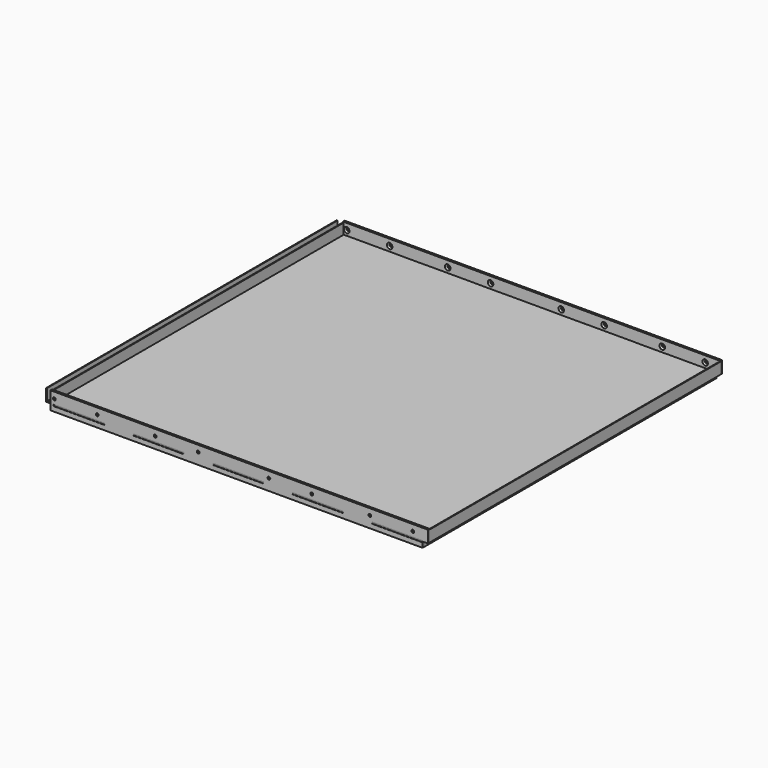
from build123d import *

# Parameters (mm, degrees)
F1_DEPTH        = 1440
F2_DEPTH        = 1440
F3_W            = 200
F3_H            = 7
F4_DEPTH        = 3
F5_W            = 200
F5_H            = 7
F6_DEPTH        = 3
F7_W            = 200.5
F7_H            = 6.5
F8_DEPTH        = 8
F11_D           = 11
F11_CSINK_D     = 22
F11_CSINK_ANGLE = 90


with BuildPart() as f1:
    # F0 (on Front) → F1 (new body)
    with BuildSketch(Plane.XZ):
        Polygon((-1400.4856245518, 88.2625505924), (-1403.4856245518, 88.2625505924), (-1403.4856245518, 40.2625505924), (91.5143754482, 40.2625505924), (91.5143754482, 21.2625505924), (94.5143754482, 21.2625505924), (94.5143754482, 43.2625505924), (-1379.4856245518, 43.2625505924), (-1400.4856245518, 43.2625505924), align=None)
    extrude(amount=-F1_DEPTH)

    # F3 (on face) → F4 (join)
    with BuildSketch(Plane.XY.offset(43.2625505924)):
        with Locations((-1266.4856245518, -3.5)):
            Rectangle(F3_W, F3_H)
        with Locations((-951.4856245518, -3.5)):
            Rectangle(F3_W, F3_H)
        with Locations((-636.4856245518, -3.5)):
            Rectangle(F3_W, F3_H)
        with Locations((-321.4856245518, -3.5)):
            Rectangle(F3_W, F3_H)
        with Locations((-6.4856245518, -3.5)):
            Rectangle(F3_W, F3_H)
        with Locations((-1266.4856245518, 1443.5)):
            Rectangle(F3_W, F3_H)
        with Locations((-951.4856245518, 1443.5)):
            Rectangle(F3_W, F3_H)
        with Locations((-321.4856245518, 1443.5)):
            Rectangle(F3_W, F3_H)
        with Locations((-6.4856245518, 1443.5)):
            Rectangle(F3_W, F3_H)
        with Locations((-636.4856245518, 1443.5)):
            Rectangle(F3_W, F3_H)
    extrude(amount=-F4_DEPTH)


with BuildPart() as f2:
    # F0 (on Front) → F2 (new body)
    with BuildSketch(Plane.XZ):
        Polygon((-1379.4856245518, 88.2625505924), (-1379.4856245518, 43.2625505924), (94.5143754482, 43.2625505924), (115.5143754482, 43.2625505924), (115.5143754482, 46.2625505924), (115.5143754482, 88.2625505924), (112.5143754482, 88.2625505924), (112.5143754482, 46.2625505924), (-1376.4856245518, 46.2625505924), (-1376.4856245518, 88.2625505924), align=None)
    extrude(amount=-F2_DEPTH)

    # F5 (on face) → F6 (join)
    with BuildSketch(Plane.XY.offset(46.2625505924)):
        with Locations((-1266.4856245518, -3.5)):
            Rectangle(F5_W, F5_H)
        with Locations((-951.4856245518, -3.5)):
            Rectangle(F5_W, F5_H)
        with Locations((-636.4856245518, -3.5)):
            Rectangle(F5_W, F5_H)
        with Locations((-321.4856245518, -3.5)):
            Rectangle(F5_W, F5_H)
        with Locations((-6.4856245518, -3.5)):
            Rectangle(F5_W, F5_H)
        with Locations((-951.4856245518, 1443.5)):
            Rectangle(F5_W, F5_H)
        with Locations((-1266.4856245518, 1443.5)):
            Rectangle(F5_W, F5_H)
        with Locations((-6.4856245518, 1443.5)):
            Rectangle(F5_W, F5_H)
        with Locations((-636.4856245518, 1443.5)):
            Rectangle(F5_W, F5_H)
        with Locations((-321.4856245518, 1443.5)):
            Rectangle(F5_W, F5_H)
    extrude(amount=-F6_DEPTH)


with BuildPart() as f8:
    # F7 (on face) → F8 (new body)
    with BuildSketch(Plane.XZ):
        Polygon((94.5143754482, 43.2625505924), (115.5143754482, 43.2625505924), (115.5143754482, 91.2625505924), (-1379.4856245518, 91.2625505924), (-1379.4856245518, 21.2625505924), (94.5143754482, 21.2625505924), align=None)
        with Locations((-1266.4856245518, 43.2625505924)):
            Rectangle(F7_W, F7_H, mode=Mode.SUBTRACT)
        with Locations((-951.4856245518, 43.2625505924)):
            Rectangle(F7_W, F7_H, mode=Mode.SUBTRACT)
        with Locations((-636.4856245518, 43.2625505924)):
            Rectangle(F7_W, F7_H, mode=Mode.SUBTRACT)
        with Locations((-321.4856245518, 43.2625505924)):
            Rectangle(F7_W, F7_H, mode=Mode.SUBTRACT)
        with Locations((-6.4856245518, 43.2625505924)):
            Rectangle(F7_W, F7_H, mode=Mode.SUBTRACT)
    extrude(amount=F8_DEPTH)

    # F11 (through all)
    with Locations(Plane(origin=(0, 0, 0), x_dir=(-1, 0, 0), z_dir=(0, 1, 0))):
        with Locations((1364.4856245518, 66.2625505924), (1194.4856245518, 66.2625505924), (964.4856245518, 66.2625505924), (794.4856245518, 66.2625505924), (514.4856245518, 66.2625505924), (344.4856245518, 66.2625505924), (114.4856245518, 66.2625505924), (-55.5143754482, 66.2625505924)):
            CounterSinkHole(F11_D / 2, F11_CSINK_D / 2, counter_sink_angle=F11_CSINK_ANGLE)


with BuildPart() as f12_1:
    # F12: instance of F8
    add(f8.part.mirror(Plane(origin=(0, 720, 0), x_dir=(-1, 0, 0), z_dir=(0, 1, 0))))


solid = Compound([f1.part, f2.part, f8.part, f12_1.part])
